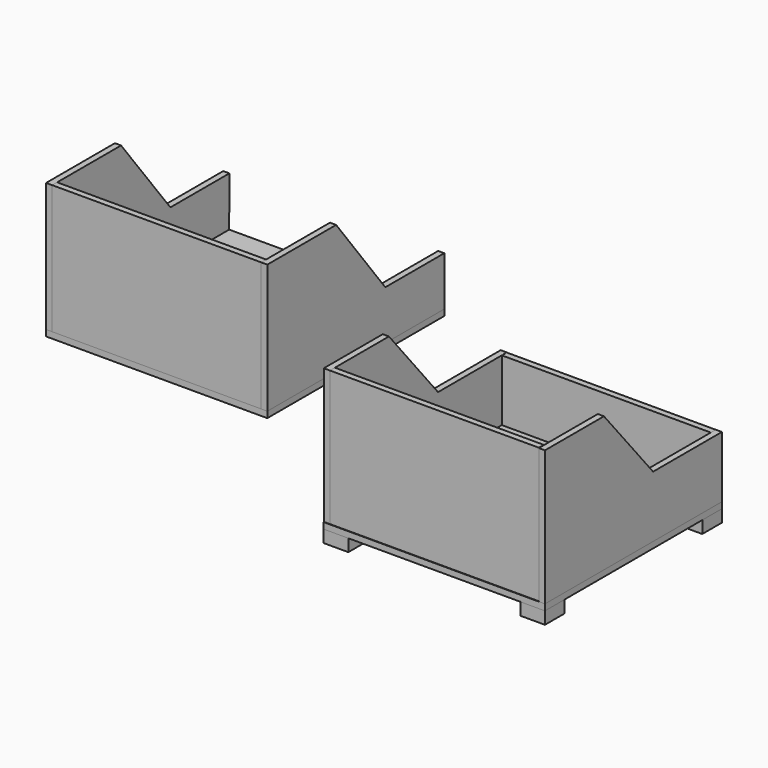
from build123d import *

# Parameters (mm, degrees)
F0_W      = 228.6
F0_H      = 228.6
F1_DEPTH  = 6.35
F2_W      = 25.4
F2_H      = 25.4
F3_DEPTH  = 12.7
F5_DEPTH  = 6.35
F7_DEPTH  = 6.35
F8_W      = 215.9
F8_H      = 63.5805330239
F9_DEPTH  = 6.35
F10_W     = 215.9
F10_H     = 139.7
F11_DEPTH = 6.35
F12_W     = 228.6
F12_H     = 228.6
F13_DEPTH = 6.35
F15_DEPTH = 6.35
F17_DEPTH = 6.35
F18_W     = 215.8993035555
F18_H     = 133.35
F19_DEPTH = 6.35


# Not quite as in the source:
# - a feature names something its author has since deleted; it is built from what else it names


with BuildPart() as f1:
    # F0 (on Top) → F1 (new body)
    with BuildSketch(Plane.XY):
        with Locations((114.3, -114.3)):
            Rectangle(F0_W, F0_H)
    extrude(amount=F1_DEPTH)


with BuildPart() as f3:
    # F2 (on face) → F3 (new body)
    with BuildSketch(Plane(origin=(0, 0, 0), x_dir=(1, 0, 0), z_dir=(0, 0, -1))):
        with Locations((12.7, 215.9)):
            Rectangle(F2_W, F2_H)
    extrude(amount=F3_DEPTH)


with BuildPart() as f3b:
    # F2 (on face) → F3, piece 2 (new body)
    with BuildSketch(Plane(origin=(0, 0, 0), x_dir=(1, 0, 0), z_dir=(0, 0, -1))):
        with Locations((215.9, 215.9)):
            Rectangle(F2_W, F2_H)
    extrude(amount=F3_DEPTH)


with BuildPart() as f3c:
    # F2 (on face) → F3, piece 3 (new body)
    with BuildSketch(Plane(origin=(0, 0, 0), x_dir=(1, 0, 0), z_dir=(0, 0, -1))):
        with Locations((12.7, 12.7)):
            Rectangle(F2_W, F2_H)
    extrude(amount=F3_DEPTH)


with BuildPart() as f3d:
    # F2 (on face) → F3, piece 4 (new body)
    with BuildSketch(Plane(origin=(0, 0, 0), x_dir=(1, 0, 0), z_dir=(0, 0, -1))):
        with Locations((215.9, 12.7)):
            Rectangle(F2_W, F2_H)
    extrude(amount=F3_DEPTH)


with BuildPart() as f5:
    # F4 (on Right) → F5 (new body)
    with BuildSketch(Plane.YZ):
        Polygon((-228.5113930702, 146.3453488544), (-228.5113930702, 6.6453488544), (0, 6.4208060503), (0, 69.9208060503), (-88.9, 69.9208060503), (-152.3113930702, 146.3453488544), align=None)
    extrude(amount=F5_DEPTH)


with BuildPart() as f7:
    # F6 (on face) → F7 (new body)
    with BuildSketch(Plane.YZ.offset(228.6)):
        Polygon((-228.6, 6.35), (0, 6.35), (0, 69.85), (-88.9, 69.85), (-152.4, 146.05), (-228.6, 146.05), align=None)
    extrude(amount=-F7_DEPTH)


with BuildPart() as f9:
    # F8 (on Front) → F9 (new body)
    with BuildSketch(Plane.XZ):
        with Locations((114.2569518656, 37.9939724226)):
            Rectangle(F8_W, F8_H)
    extrude(amount=F9_DEPTH)


with BuildPart() as f11:
    # F10 (on face) → F11 (new body)
    with BuildSketch(Plane.XZ.offset(228.5113930702)):
        with Locations((114.3, 76.4953488544)):
            Rectangle(F10_W, F10_H)
    extrude(amount=-F11_DEPTH)


with BuildPart() as f13:
    # F12 (on Top) → F13 (new body)
    with BuildSketch(Plane.XY):
        with Locations((-270.9899397628, 8.6805075407)):
            Rectangle(F12_W, F12_H)
    extrude(amount=F13_DEPTH)


with BuildPart() as f15:
    # F14 (on face) → F15 (new body)
    with BuildSketch(Plane(origin=(-385.2899397628, 0, 0), x_dir=(0, -1, 0), z_dir=(-1, 0, 0))):
        Polygon((-46.9879293919, 57.4492700398), (-123.1879293919, 57.4492700398), (-122.9805075407, 6.35), (105.6194924593, 6.35), (105.6194924593, 139.7), (16.7194924593, 139.7), align=None)
    extrude(amount=-F15_DEPTH)


with BuildPart() as f17:
    # F16 (on face) → F17 (new body)
    with BuildSketch(Plane.YZ.offset(-156.6899397628)):
        Polygon((-105.6194924593, 6.35), (122.9805075407, 6.35), (122.9805075407, 57.15), (46.7805075407, 57.15), (-16.7194924593, 139.7), (-105.6194924593, 139.7), align=None)
    extrude(amount=-F17_DEPTH)


with BuildPart() as f19:
    # F18 (on face) → F19 (new body)
    with BuildSketch(Plane.XZ.offset(105.6194924593)):
        with Locations((-270.9895297885, 73.025)):
            Rectangle(F18_W, F18_H)
    extrude(amount=-F19_DEPTH)


solid = Compound([f1.part, f3.part, f3b.part, f3c.part, f3d.part, f5.part, f7.part, f9.part, f11.part, f13.part, f15.part, f17.part, f19.part])
